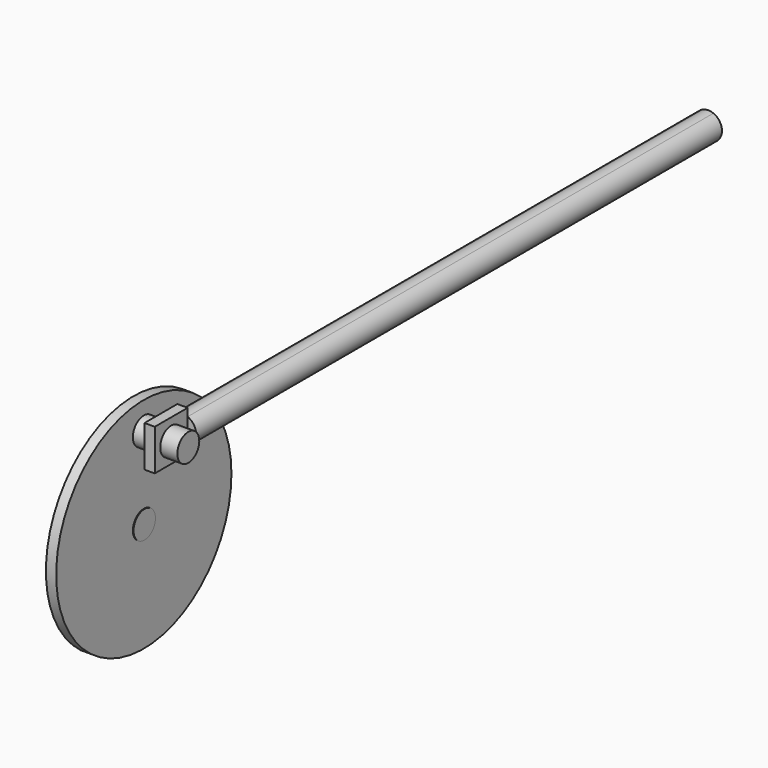
from build123d import *

# Parameters (mm, degrees)
F0_R          = 50.8
F0_R_2        = 6.35
F1_DEPTH      = 4.7625
F2_DEPTH      = 25.4
F4_W          = 19.05
F4_H          = 19.05
F5_DEPTH      = 4.7625
F7_DEPTH      = 304.8
F8_DEPTH      = 25.4
F8_DEPTH_BACK = 5.08


# Not quite as in the source:
# - a feature names something its author has since deleted; it is built from what else it names


with BuildPart() as f1:
    # F0 (on Right) → F1 (new body)
    with BuildSketch(Plane.YZ):
        Circle(F0_R)
        Circle(F0_R_2, mode=Mode.SUBTRACT)
        with Locations((0, 38.1)):
            Circle(F0_R_2, mode=Mode.SUBTRACT)
    extrude(amount=F1_DEPTH)


with BuildPart() as f2:
    # F0 (on Right) → F2 (new body)
    with BuildSketch(Plane.YZ):
        with Locations((0, 38.1)):
            Circle(F0_R_2)
    extrude(amount=F2_DEPTH)


with BuildPart() as f5:
    # F4 (on offset) → F5 (new body)
    with BuildSketch(Plane.YZ.offset(12.7)):
        with Locations((0, 38.2848121226)):
            Rectangle(F4_W, F4_H)
    extrude(amount=F5_DEPTH)

    # F6 (on face) → F7 (join)
    with BuildSketch(Plane(origin=(0, 9.525, 0), x_dir=(-1, 0, 0), z_dir=(0, 1, 0))):
        with BuildLine():
            Line((-17.4625, 32.3982045735), (-17.4625, 44.1714196717))
            ThreePointArc((-17.4625, 44.1714196717), (-21.43125, 38.2848121226), (-17.4625, 32.3982045735))
        make_face()
        with BuildLine():
            Line((-12.7, 32.3982045735), (-12.7, 44.1714196717))
            ThreePointArc((-12.7, 44.1714196717), (-15.08125, 44.6348121226), (-17.4625, 44.1714196717))
            Line((-17.4625, 44.1714196717), (-17.4625, 32.3982045735))
            ThreePointArc((-17.4625, 32.3982045735), (-15.08125, 31.9348121226), (-12.7, 32.3982045735))
        make_face()
        with BuildLine():
            ThreePointArc((-12.7, 32.3982045735), (-9.8161081453, 34.7350542083), (-8.73125, 38.2848121226))
            ThreePointArc((-8.73125, 38.2848121226), (-9.8161081453, 41.8345700369), (-12.7, 44.1714196717))
            Line((-12.7, 44.1714196717), (-12.7, 32.3982045735))
        make_face()
    extrude(amount=F7_DEPTH)


with BuildPart() as f8:
    # F0 (on Right) → F8 (new body, two sides)
    with BuildSketch(Plane.YZ) as f8_sk:
        Circle(F0_R_2)
    extrude(amount=-F8_DEPTH)
    extrude(f8_sk.sketch, amount=F8_DEPTH_BACK)


solid = Compound([f1.part, f2.part, f5.part, f8.part])
